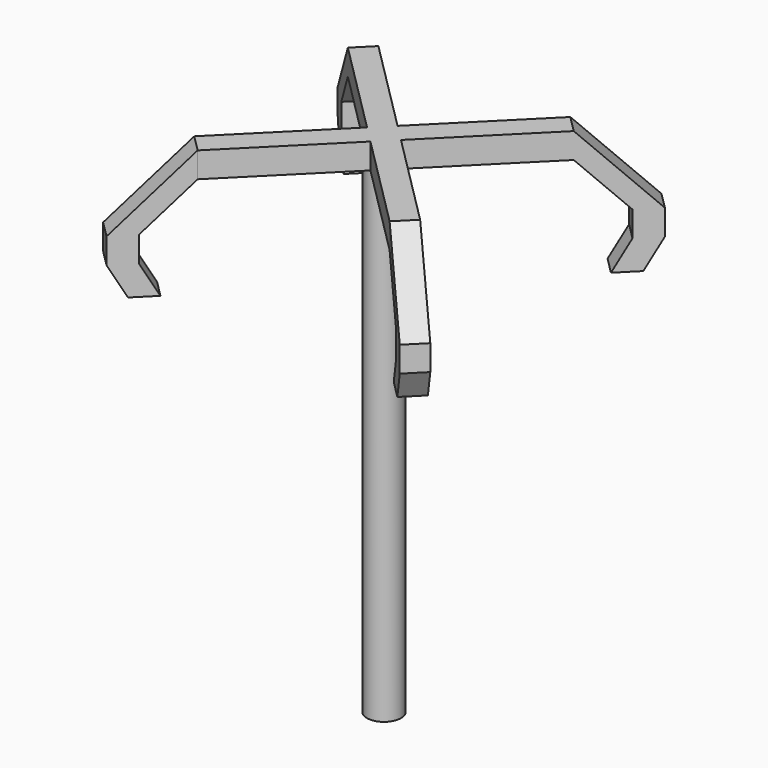
from build123d import *

# Parameters (mm, degrees)
F0_R     = 10
F1_DEPTH = 300
F3_DEPTH = 15
F5_DEPTH = 14.142


# Not quite as in the source:
# - a feature of the source that left no trace in its solid (it failed there, or was rolled back) is left out


with BuildPart() as f1:
    # F0 (on Top) → F1 (new body)
    with BuildSketch(Plane.XY):
        Circle(F0_R)
    extrude(amount=F1_DEPTH)

    # F2 (on face) → F3 (join)
    with BuildSketch(Plane.XY.offset(300)):
        Polygon((10, 0), (10, 10), (0, 10), (-10, 10), (-10, 0), (-10, -10), (0, -10), (10, -10), align=None)
        Polygon((0, 10), (10, 10), (10, 0), (66.5685424949, 56.5685424949), (56.5685424949, 66.5685424949), align=None)
        Polygon((-10, 10), (0, 10), (-56.5685424949, 66.5685424949), (-66.5685424949, 56.5685424949), (-10, 0), align=None)
        Polygon((66.5685424949, -56.5685424949), (10, 0), (10, -10), (0, -10), (56.5685424949, -66.5685424949), align=None)
        Polygon((-10, -10), (-10, 0), (-66.5685424949, -56.5685424949), (-56.5685424949, -66.5685424949), (0, -10), align=None)
    extrude(amount=-F3_DEPTH)

    # F4 (on face) → F5 (join)
    with BuildSketch(Plane(origin=(5, -5, 0), x_dir=(0.7071067812, 0.7071067812, 0), z_dir=(0.7071067812, -0.7071067812, 0))):
        Polygon((129.2763065782, 257.7947612337), (87.0710678119, 300), (87.0710678119, 285), (114.2763065782, 257.7947612337), (114.2763065782, 242.7947612337), (129.2763065782, 242.7947612337), align=None)
        Polygon((119.3018365804, 225.5184724189), (129.2763065782, 242.7947612337), (114.2763065782, 242.7947612337), (104.3018365804, 225.5184724189), align=None)
    extrude(amount=-F5_DEPTH)

    # F6: F1 across plane


with BuildPart() as f1_1:
    add(f1.part)
    add(f1.part.mirror(Plane.XZ))

    # F7: F1 across plane


with BuildPart() as f1_2:
    add(f1_1.part)
    add(f1_1.part.mirror(Plane.YZ))


solid = f1_2.part
